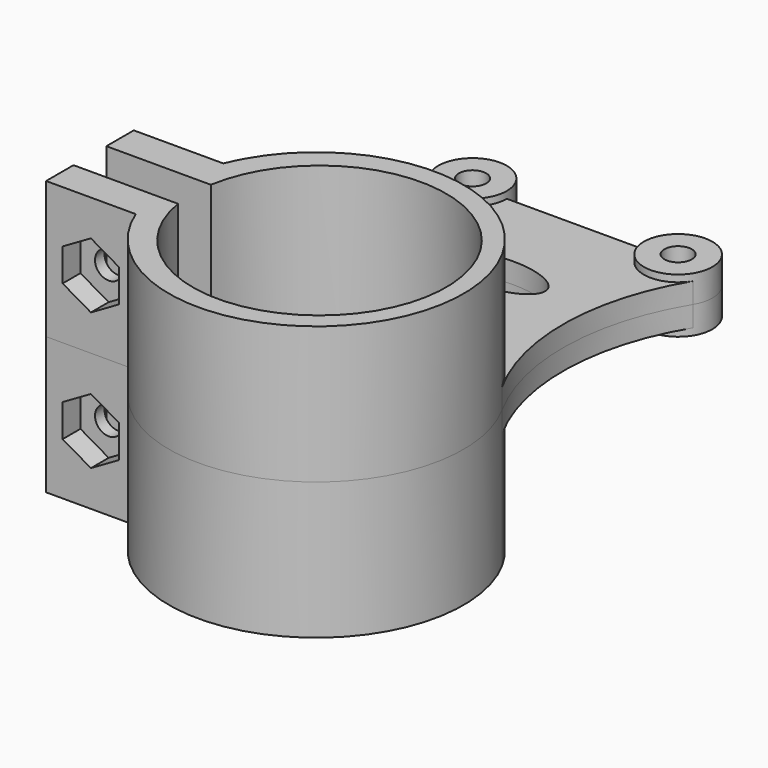
from build123d import *

# Parameters (mm, degrees)
F1_DEPTH = 20
F0_R     = 2
F2_DEPTH = 3
F3_DEPTH = 4
F5_DEPTH = 3.25
F6_R     = 2
F7_DEPTH = 29.5010001


# Not quite as in the source:
# - a feature names something its author has since deleted; it is built from what else it names


with BuildPart() as f1:
    # F0 (on Top) → F1 (new body)
    with BuildSketch(Plane.XY):
        with BuildLine():
            ThreePointArc((-18.2551362635, 3.1646558729), (18.5, 0.1646558729), (-18.2551362635, -2.8353441271))
            Line((-18.2551362635, -2.8353441271), (-21.289668856, -2.8353441271))
            Line((-21.289668856, -2.8353441271), (-33.5, -2.8353441271))
            Line((-33.5, -2.8353441271), (-33.5, -5.8353441271))
            Line((-33.5, -5.8353441271), (-33.5, -7.8353441271))
            Line((-33.5, -7.8353441271), (-20.4217309456, -7.8353441271))
            ThreePointArc((-20.4217309456, -7.8353441271), (8.7176252261, -19.2755005117), (18.3885107603, 10.4978639134))
            ThreePointArc((18.3885107603, 10.4978639134), (-0.3478610365, 21.6643338769), (-19.2053350681, 10.7036152553))
            ThreePointArc((-19.2053350681, 10.7036152553), (-19.8551354356, 9.4540669672), (-20.4217309456, 8.1646558729))
            Line((-20.4217309456, 8.1646558729), (-33.5, 8.1646558729))
            Line((-33.5, 8.1646558729), (-33.5, 6.1646558729))
            Line((-33.5, 6.1646558729), (-33.5, 3.1646558729))
            Line((-33.5, 3.1646558729), (-21.289668856, 3.1646558729))
            Line((-21.289668856, 3.1646558729), (-18.2551362635, 3.1646558729))
        make_face()
    extrude(amount=F1_DEPTH)

    # F0 (on Top) → F2 (join)
    with BuildSketch(Plane.XY):
        with BuildLine():
            ThreePointArc((-19.2053350681, 10.7036152553), (-0.3478610365, 21.6643338769), (18.3885107603, 10.4978639134))
            ThreePointArc((18.3885107603, 10.4978639134), (14.2120337074, 27.5685018888), (19.1172770705, 44.4441716239))
            ThreePointArc((19.1172770705, 44.4441716239), (13.4958098431, 42.2172179553), (9.8397882001, 47.0332040616))
            Line((9.8397882001, 47.0332040616), (-10.1602117999, 47.0332040616))
            ThreePointArc((-10.1602117999, 47.0332040616), (-13.8544265436, 42.2067224379), (-19.4781817457, 44.512264644))
            ThreePointArc((-19.4781817457, 44.512264644), (-14.8414845345, 27.6442586076), (-19.2053350681, 10.7036152553))
        make_face()
        with BuildLine():
            add(Edge.make_bspline(
                [(7.5, 31.9373905659), (7.5, 37.9995683924), (-3.75, 34.9684794791), (-15, 31.9373905659), (-3.75, 28.9063016526), (7.5, 25.8752127394), (7.5, 31.9373905659)],
                knots=[0, 0, 0, 2.0943951024, 2.0943951024, 4.1887902048, 4.1887902048, 6.2831853072, 6.2831853072, 6.2831853072], degree=2, weights=[1, 0.5, 1, 0.5, 1, 0.5, 1]))
        make_face(mode=Mode.SUBTRACT)
        with BuildLine():
            ThreePointArc((-10.1602117999, 47.0332040616), (-16.4659970562, 51.8596856854), (-19.4781817457, 44.512264644))
            ThreePointArc((-19.4781817457, 44.512264644), (-13.8544265436, 42.2067224379), (-10.1602117999, 47.0332040616))
        make_face()
        with Locations((-15.1602117999, 47.0332040616)):
            Circle(F0_R, mode=Mode.SUBTRACT)
        with BuildLine():
            ThreePointArc((9.8397882001, 47.0332040616), (13.4958098431, 42.2172179553), (19.1172770705, 44.4441716239))
            ThreePointArc((19.1172770705, 44.4441716239), (19.6557743064, 45.6892257046), (19.8397882001, 47.0332040616))
            ThreePointArc((19.8397882001, 47.0332040616), (14.8397882001, 52.0332040616), (9.8397882001, 47.0332040616))
        make_face()
        with BuildLine():
            ThreePointArc((16.8397882001, 47.0332040616), (14.8397882001, 45.0332040616), (12.8397882001, 47.0332040616))
            ThreePointArc((12.8397882001, 47.0332040616), (14.8397882001, 49.0332040616), (16.8397882001, 47.0332040616))
        make_face(mode=Mode.SUBTRACT)
    extrude(amount=F2_DEPTH)

    # F0 (on Top) → F3 (join)
    with BuildSketch(Plane.XY):
        with BuildLine():
            ThreePointArc((-10.1602117999, 47.0332040616), (-16.4659970562, 51.8596856854), (-19.4781817457, 44.512264644))
            ThreePointArc((-19.4781817457, 44.512264644), (-13.8544265436, 42.2067224379), (-10.1602117999, 47.0332040616))
        make_face()
        with Locations((-15.1602117999, 47.0332040616)):
            Circle(F0_R, mode=Mode.SUBTRACT)
        with BuildLine():
            ThreePointArc((9.8397882001, 47.0332040616), (13.4958098431, 42.2172179553), (19.1172770705, 44.4441716239))
            ThreePointArc((19.1172770705, 44.4441716239), (19.6557743064, 45.6892257046), (19.8397882001, 47.0332040616))
            ThreePointArc((19.8397882001, 47.0332040616), (14.8397882001, 52.0332040616), (9.8397882001, 47.0332040616))
        make_face()
        with BuildLine():
            ThreePointArc((16.8397882001, 47.0332040616), (14.8397882001, 45.0332040616), (12.8397882001, 47.0332040616))
            ThreePointArc((12.8397882001, 47.0332040616), (14.8397882001, 49.0332040616), (16.8397882001, 47.0332040616))
        make_face(mode=Mode.SUBTRACT)
    extrude(amount=F3_DEPTH)

    # F4 (on face) → F5 (cut)
    with BuildSketch(Plane.XZ.offset(7.8353441271)):
        Polygon((-31.0858654728, 12.3815698604), (-31.0858654728, 7.6184301396), (-26.9608654728, 5.2368602792), (-22.8358654728, 7.6184301396), (-22.8358654728, 12.3815698604), (-26.9608654728, 14.7631397208), align=None)
    extrude(amount=-F5_DEPTH, mode=Mode.SUBTRACT)

    # F6 (on face) → F7 (cut, through all)
    with BuildSketch(Plane(origin=(0, 8.1646558729, 0), x_dir=(-1, 0, 0), z_dir=(0, 1, 0))):
        with Locations((26.9608654728, 10)):
            Circle(F6_R)
    extrude(amount=-F7_DEPTH, mode=Mode.SUBTRACT)


with BuildPart() as f8_1:
    # F8: instance of F1
    add(f1.part.mirror(Plane.XY))


solid = Compound([f1.part, f8_1.part])
